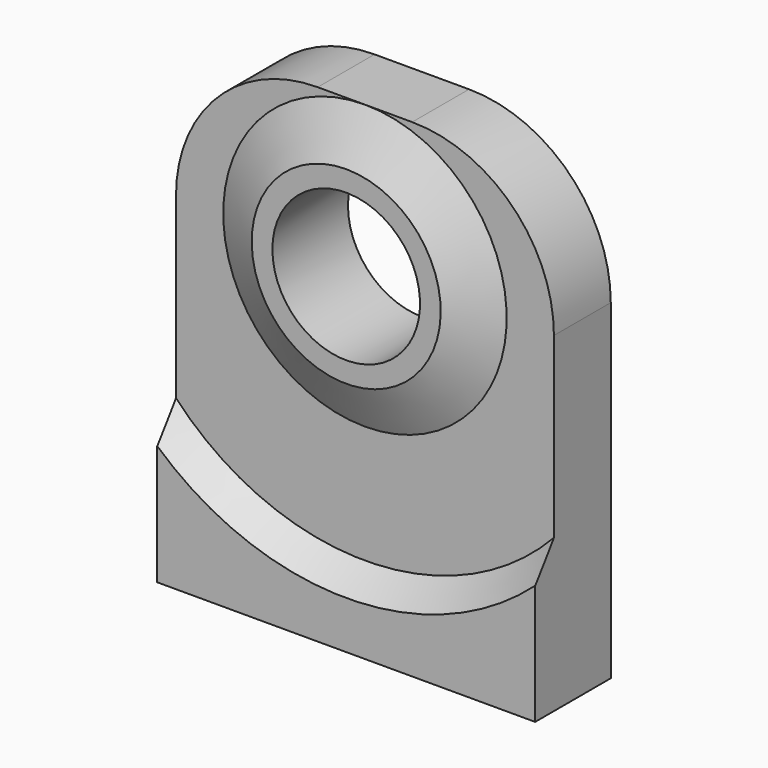
from build123d import *

# Parameters (mm, degrees)
F0_R     = 4.953
F1_DEPTH = 4.7752
F2_DEPTH = 6.35
F4_DEPTH = 1.5748
F5_SIZE2 = 1.57479
F5_SIZE  = 3.17499
F6_SIZE  = 1.57479
F7_R     = 9.525
F8_R     = 4.953
F9_DEPTH = 6.35
F11_D    = 9.92124


# Not quite as in the source:
# - a fillet or chamfer is up to 0.001 mm smaller than in the source, because OpenCascade refuses the exact size


with BuildPart() as f1:
    # F0 (on Front) → F1 (new body)
    with BuildSketch(Plane.XZ):
        Polygon((0, 31.75), (0, 0), (25.4, 0), (25.4, 31.75), (12.7, 31.75), align=None)
        with BuildLine():
            ThreePointArc((22.225, 22.225), (5.9648079092, 15.4898079092), (12.7, 31.75))
            ThreePointArc((12.7, 31.75), (19.4351920908, 28.9601920908), (22.225, 22.225))
        make_face(mode=Mode.SUBTRACT)
        with BuildLine():
            ThreePointArc((22.225, 22.225), (19.4351920908, 28.9601920908), (12.7, 31.75))
            ThreePointArc((12.7, 31.75), (5.9648079092, 15.4898079092), (22.225, 22.225))
        make_face()
        with Locations((12.7, 22.225)):
            Circle(F0_R, mode=Mode.SUBTRACT)
    extrude(amount=F1_DEPTH)

    # F0 (on Front) → F2 (join)
    with BuildSketch(Plane.XZ):
        with BuildLine():
            ThreePointArc((22.225, 22.225), (19.4351920908, 28.9601920908), (12.7, 31.75))
            ThreePointArc((12.7, 31.75), (5.9648079092, 15.4898079092), (22.225, 22.225))
        make_face()
        with Locations((12.7, 22.225)):
            Circle(F0_R, mode=Mode.SUBTRACT)
    extrude(amount=F2_DEPTH)

    # F3 (on face) → F4 (join, through all)
    with BuildSketch(Plane.XZ.offset(6.35)):
        with BuildLine():
            ThreePointArc((25.4, 10.2581491177), (12.7, 4.7752), (0, 10.2581491177))
            Line((0, 10.2581491177), (0, 0))
            Line((0, 0), (25.4, 0))
            Line((25.4, 0), (25.4, 10.2581491177))
        make_face()
    extrude(amount=-F4_DEPTH)

    # F5 (size 3.175 and 1.5748 in the source; OpenCascade refuses exactly that, so slightly less here)
    f5_edges = [f1.edges().sort_by_distance(p)[0] for p in [
        (3.175, -6.35, 22.225),
    ]]
    f5_side = f1.faces().sort_by_distance((3.444408, -6.35, 22.225))[0]
    chamfer(f5_edges, length=F5_SIZE, length2=F5_SIZE2, reference=f5_side)

    # F6 (size 1.5748 in the source; OpenCascade refuses exactly that, so slightly less here)
    f6_edges = [f1.edges().sort_by_distance(p)[0] for p in [
        (12.7, -6.35, 4.7752),
    ]]
    chamfer(f6_edges, length=F6_SIZE)

    # F7
    f7_edges = [f1.edges().sort_by_distance(p)[0] for p in [
        (0, -2.3876, 31.75),
        (25.4, -2.3876, 31.75),
    ]]
    fillet(f7_edges, radius=F7_R)

    # F8 (on face) → F9 (join, through all)
    with BuildSketch(Plane.XZ.offset(6.35)):
        with Locations((12.7, 22.225)):
            Circle(F8_R)
    extrude(amount=-F9_DEPTH)

    # F11 (through all)
    with Locations(Plane.XZ.offset(6.35)):
        with Locations((12.7, 22.225)):
            Hole(F11_D / 2)


solid = f1.part
